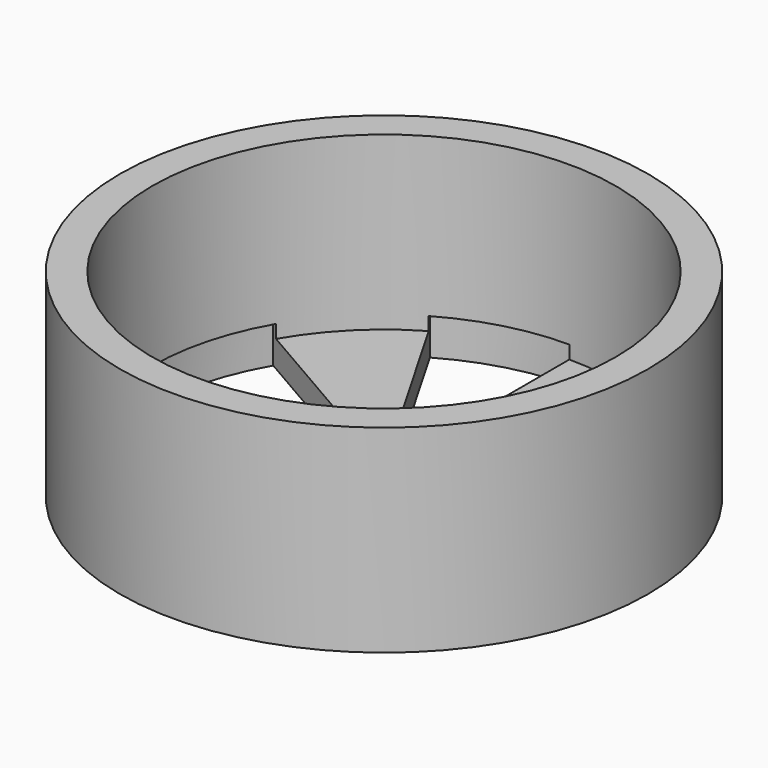
from build123d import *

# Parameters (mm, degrees)
F0_R     = 20
F1_DEPTH = 15
F2_R     = 17.5460358756
F4_DEPTH = 13
F6_DEPTH = 3


# Not quite as in the source:
# - a feature of the source that left no trace in its solid (it failed there, or was rolled back) is left out


with BuildPart() as f1:
    # F0 (on Top) → F1 (new body)
    with BuildSketch(Plane.XY):
        Circle(F0_R)
    extrude(amount=F1_DEPTH)

    # F2 (on face) → F4 (cut)
    with BuildSketch(Plane.XY.offset(15)):
        Circle(F2_R)
    extrude(amount=-F4_DEPTH, mode=Mode.SUBTRACT)

    # F5 (on face) → F6 (cut)
    with BuildSketch(Plane.XY):
        with BuildLine():
            ThreePointArc((0, -18), (4.6587428118, -17.3866648732), (9, -15.5884572681))
            Line((9, -15.5884572681), (1.75, -3.0310889132))
            ThreePointArc((1.75, -3.0310889132), (0.9058666579, -3.380740392), (0, -3.5))
            Line((0, -3.5), (0, -18))
        make_face()
        with BuildLine():
            ThreePointArc((15.5884572681, -9), (17.3866648732, -4.6587428118), (18, 0))
            Line((18, 0), (3.5, 0))
            ThreePointArc((3.5, 0), (3.380740392, -0.9058666579), (3.0310889132, -1.75))
            Line((3.0310889132, -1.75), (15.5884572681, -9))
        make_face()
        with BuildLine():
            Line((3.0310889132, 1.75), (15.5884572681, 9))
            ThreePointArc((15.5884572681, 9), (12.7279220614, 12.7279220614), (9, 15.5884572681))
            Line((9, 15.5884572681), (1.75, 3.0310889132))
            ThreePointArc((1.75, 3.0310889132), (2.4748737342, 2.4748737342), (3.0310889132, 1.75))
        make_face()
        with BuildLine():
            Line((0, 3.5), (0, 18))
            ThreePointArc((0, 18), (-4.6587428118, 17.3866648732), (-9, 15.5884572681))
            Line((-9, 15.5884572681), (-1.75, 3.0310889132))
            ThreePointArc((-1.75, 3.0310889132), (-0.9058666579, 3.380740392), (0, 3.5))
        make_face()
        with BuildLine():
            Line((-3.0310889132, 1.75), (-15.5884572681, 9))
            ThreePointArc((-15.5884572681, 9), (-17.3866648732, 4.6587428118), (-18, 0))
            Line((-18, 0), (-3.5, 0))
            ThreePointArc((-3.5, 0), (-3.380740392, 0.9058666579), (-3.0310889132, 1.75))
        make_face()
        with BuildLine():
            ThreePointArc((-15.5884572681, -9), (-12.7279220614, -12.7279220614), (-9, -15.5884572681))
            Line((-9, -15.5884572681), (-1.75, -3.0310889132))
            ThreePointArc((-1.75, -3.0310889132), (-2.4748737342, -2.4748737342), (-3.0310889132, -1.75))
            Line((-3.0310889132, -1.75), (-15.5884572681, -9))
        make_face()
    extrude(amount=F6_DEPTH, mode=Mode.SUBTRACT)


solid = f1.part
